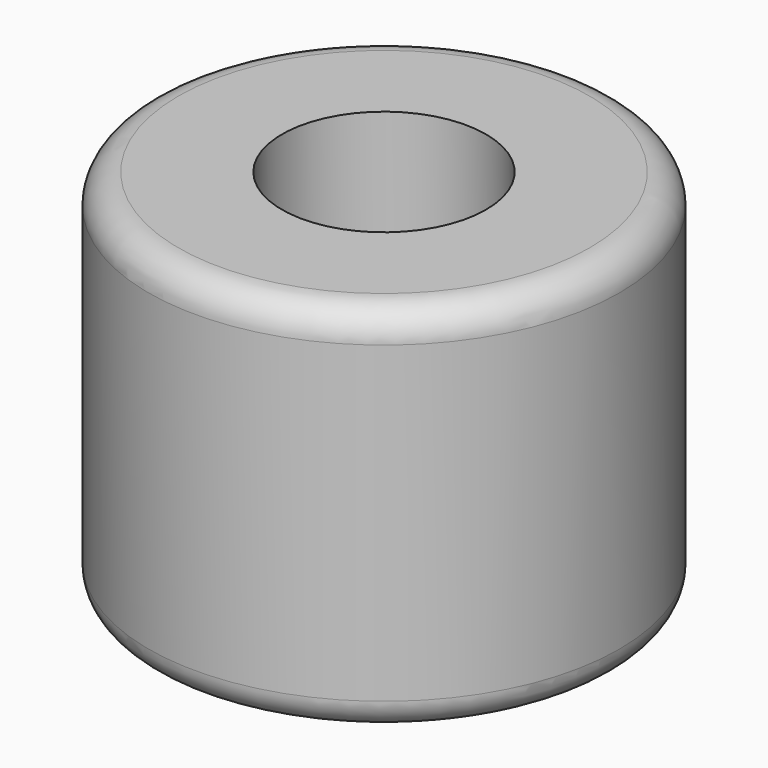
from build123d import *

# Parameters (mm, degrees)
F0_R     = 15.7692613996
F1_DEPTH = 25
F2_R     = 2
F3_R     = 6.8344152612
F4_DEPTH = 40


# Not quite as in the source:
# - a feature names something its author has since deleted; it is built from what else it names


with BuildPart() as f1:
    # F0 (on Top) → F1 (new body)
    with BuildSketch(Plane.XY):
        with Locations((-22.6599406451, -18.1141793728)):
            Circle(F0_R)
    extrude(amount=F1_DEPTH)

    # F2
    f2_edges = [f1.edges().sort_by_distance(p)[0] for p in [
        (-38.429202, -18.114179, 0),
        (-38.429202, -18.114179, 25),
    ]]
    fillet(f2_edges, radius=F2_R)

    # F3 (on face) → F4 (cut)
    with BuildSketch(Plane(origin=(0, 0, 0), x_dir=(1, 0, 0), z_dir=(0, 0, -1))):
        with Locations((-22.6599406451, 18.1141793728)):
            Circle(F3_R)
    extrude(amount=-F4_DEPTH, mode=Mode.SUBTRACT)


solid = f1.part
